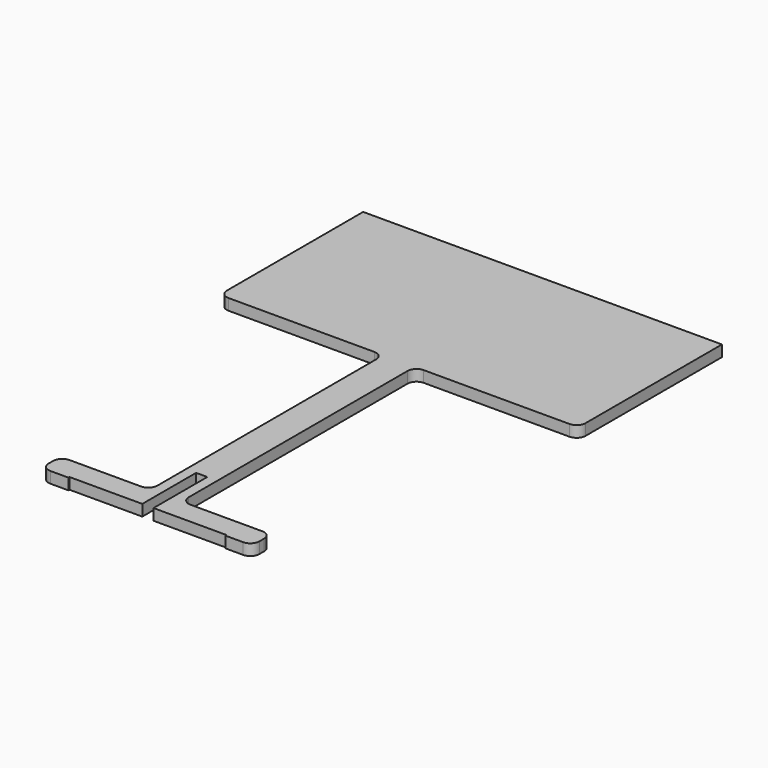
from build123d import *

# Parameters (mm, degrees)
F0_W     = 6
F0_H     = 0.3
F1_DEPTH = 2.5
F2_R     = 2


# Not quite as in the source:
# - a feature names something its author has since deleted; it is built from what else it names


with BuildPart() as f1:
    # F0 (on Top) → F1 (new body)
    with BuildSketch(Plane.XY):
        Polygon((3.5, 0), (-3.5, 0), (-3.5, -65), (-23.5, -65), (-23.5, -70), (-17.5, -70), (-1.25, -70), (-1.25, -55), (1.25, -55), (1.25, -70), (17.5, -70), (23.5, -70), (23.5, -65), (3.5, -65), align=None)
        with Locations((-20.5, -70.15)):
            Rectangle(F0_W, F0_H)
        with Locations((20.5, -70.15)):
            Rectangle(F0_W, F0_H)
        Polygon((-40, 40), (-40, 0), (-3.5, 0), (3.5, 0), (40, 0), (40, 40), align=None)
    extrude(amount=F1_DEPTH)

    # F2
    f2_edges = [f1.edges().sort_by_distance(p)[0] for p in [
        (-3.5, 0, 1.25),
        (3.5, 0, 1.25),
        (3.5, -65, 1.25),
        (-3.5, -65, 1.25),
        (-23.5, -65, 1.25),
        (23.5, -65, 1.25),
        (-23.5, -70.3, 1.25),
        (23.5, -70.3, 1.25),
        (40, 0, 1.25),
        (-40, 0, 1.25),
    ]]
    fillet(f2_edges, radius=F2_R)


solid = f1.part
